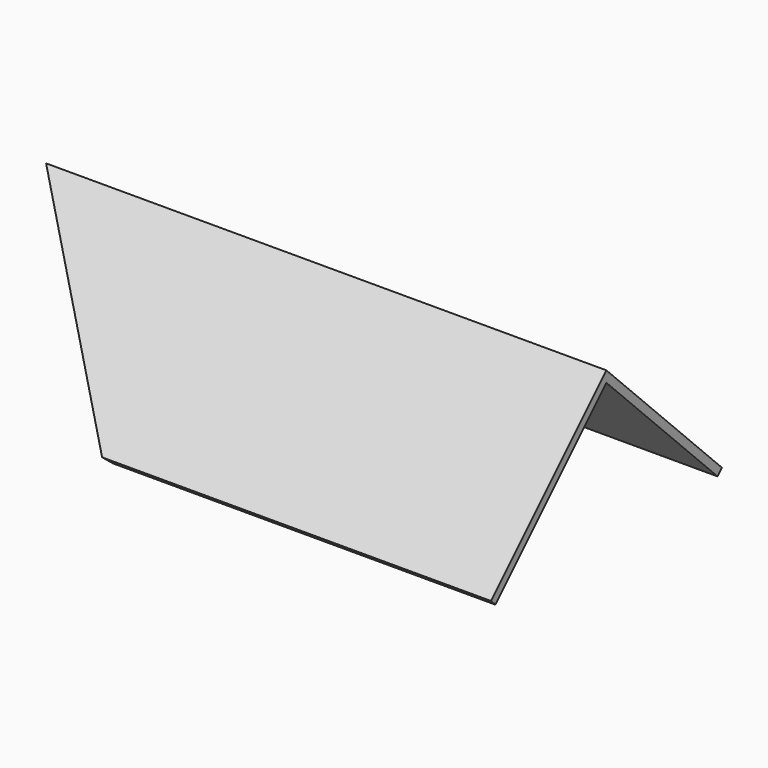
from build123d import *

# Parameters (mm, degrees)
F1_DEPTH  = 247.3
F3_DEPTH  = 300
F4_DEPTH  = 50
F5_DEPTH  = 59.1
F6_DEPTH  = 300
F7_DEPTH  = 300
F8_DEPTH  = 17.109
F9_DEPTH  = 1.9
F10_DEPTH = 1
F11_DEPTH = 3


with BuildPart() as f1:
    # F0 (on Front) → F1 (new body)
    with BuildSketch(Plane.XZ):
        Polygon((-78.8866152354, 43.4383174348), (-78.6296018241, 42.9628188217), (-78.6296018241, 102.819841868), (-127.7663317061, 102.819841868), (-96.9769939736, 76.9071934711), align=None)
        Polygon((-79.7663317061, 42.9628188217), (-97.7663317061, 76.264485822), (-127.7663317061, 101.5128188217), (-157.7663317061, 76.264485822), (-175.7663317061, 42.9628188217), align=None)
        Polygon((-127.7663317061, 101.5128188217), (-97.7663317061, 76.264485822), (-79.7663317061, 42.9628188217), (-78.6296018241, 42.9628188217), (-78.8866152354, 43.4383174348), (-96.9769939736, 76.9071934711), (-127.7663317061, 102.819841868), (-158.5556694386, 76.9071934711), (-176.9030615881, 42.9628188217), (-175.7663317061, 42.9628188217), (-157.7663317061, 76.264485822), align=None)
        Polygon((-176.9030615881, 102.819841868), (-176.9030615881, 42.9628188217), (-158.5556694386, 76.9071934711), (-127.7663317061, 102.819841868), align=None)
    extrude(amount=-F1_DEPTH)

    # F0 (on Front) → F3 (cut)
    with BuildSketch(Plane.XZ):
        Polygon((-78.8866152354, 43.4383174348), (-78.6296018241, 42.9628188217), (-78.6296018241, 102.819841868), (-127.7663317061, 102.819841868), (-96.9769939736, 76.9071934711), align=None)
    extrude(amount=-F3_DEPTH, mode=Mode.SUBTRACT)

    # F2 (on face) → F4 (join)
    with BuildSketch(Plane.YZ.offset(-78.6296018241)):
        Polygon((142.2357864376, 84.2340554304), (123.65, 102.819841868), (123.65, 101.4056283057), (141.5286796564, 83.5269486492), align=None)
        Polygon((123.65, 101.4056283057), (123.65, 102.819841868), (105.0642135624, 84.2340554304), (105.7713203436, 83.5269486492), align=None)
    extrude(amount=-F4_DEPTH)

    # F2 (on face) → F5 (join)
    with BuildSketch(Plane.YZ.offset(-78.6296018241)):
        Polygon((103.65, 42.9628188217), (123.65, 42.9628188217), (123.65, 82.819841868), (106.4784271247, 82.819841868), (105.0642135624, 82.819841868), (103.65, 82.819841868), align=None)
        Polygon((123.65, 42.9628188217), (143.65, 42.9628188217), (143.65, 82.819841868), (142.2357864376, 82.819841868), (140.8215728753, 82.819841868), (123.65, 82.819841868), align=None)
    extrude(amount=-F5_DEPTH)

    # F2 (on face) → F6 (cut)
    with BuildSketch(Plane.YZ.offset(-78.6296018241)):
        Polygon((247.3, 42.9628188217), (247.3, 102.819841868), (123.65, 102.819841868), (142.2357864376, 84.2340554304), (141.5286796564, 83.5269486492), (142.2357864376, 82.819841868), (143.65, 82.819841868), (143.65, 42.9628188217), align=None)
        Polygon((105.0642135624, 84.2340554304), (123.65, 102.819841868), (0, 102.819841868), (0, 42.9628188217), (103.65, 42.9628188217), (103.65, 82.819841868), (105.0642135624, 82.819841868), (105.7713203436, 83.5269486492), align=None)
        Polygon((123.65, 42.9628188217), (143.65, 42.9628188217), (143.65, 82.819841868), (142.2357864376, 82.819841868), (140.8215728753, 82.819841868), (123.65, 82.819841868), align=None)
        Polygon((103.65, 42.9628188217), (123.65, 42.9628188217), (123.65, 82.819841868), (106.4784271247, 82.819841868), (105.0642135624, 82.819841868), (103.65, 82.819841868), align=None)
    extrude(amount=-F6_DEPTH, mode=Mode.SUBTRACT)

    # F0 (on Front) → F7 (cut)
    with BuildSketch(Plane.XZ):
        Polygon((-176.9030615881, 102.819841868), (-176.9030615881, 42.9628188217), (-158.5556694386, 76.9071934711), (-127.7663317061, 102.819841868), align=None)
        Polygon((-127.7663317061, 101.5128188217), (-97.7663317061, 76.264485822), (-79.7663317061, 42.9628188217), (-78.6296018241, 42.9628188217), (-78.8866152354, 43.4383174348), (-96.9769939736, 76.9071934711), (-127.7663317061, 102.819841868), (-158.5556694386, 76.9071934711), (-176.9030615881, 42.9628188217), (-175.7663317061, 42.9628188217), (-157.7663317061, 76.264485822), align=None)
        Polygon((-79.7663317061, 42.9628188217), (-97.7663317061, 76.264485822), (-127.7663317061, 101.5128188217), (-157.7663317061, 76.264485822), (-175.7663317061, 42.9628188217), align=None)
    extrude(amount=-F7_DEPTH, mode=Mode.SUBTRACT)

    # F2 (on face) → F8 (join)
    with BuildSketch(Plane.YZ.offset(-78.6296018241)):
        Polygon((123.65, 101.4056283057), (123.65, 102.819841868), (105.0642135624, 84.2340554304), (105.7713203436, 83.5269486492), align=None)
        Polygon((142.2357864376, 84.2340554304), (123.65, 102.819841868), (123.65, 101.4056283057), (141.5286796564, 83.5269486492), align=None)
    extrude(amount=F8_DEPTH)

    # F9 (add): a face of the model
    f9_faces = [f1.faces().sort_by_distance(p)[0] for p in [
        (-61.5206018241, 114.6532437055, 93.2308117249),
    ]]
    extrude(f9_faces, amount=F9_DEPTH)

    # F10 (add): a face of the model
    f10_faces = [f1.faces().sort_by_distance(p)[0] for p in [
        (-59.6206018241, 114.6532437055, 93.2308117249),
    ]]
    extrude(f10_faces, amount=F10_DEPTH)

    # F11 (add): a face of the model
    f11_faces = [f1.faces().sort_by_distance(p)[0] for p in [
        (-58.6206018241, 114.6532437055, 93.2308117249),
    ]]
    extrude(f11_faces, amount=F11_DEPTH)


solid = f1.part
